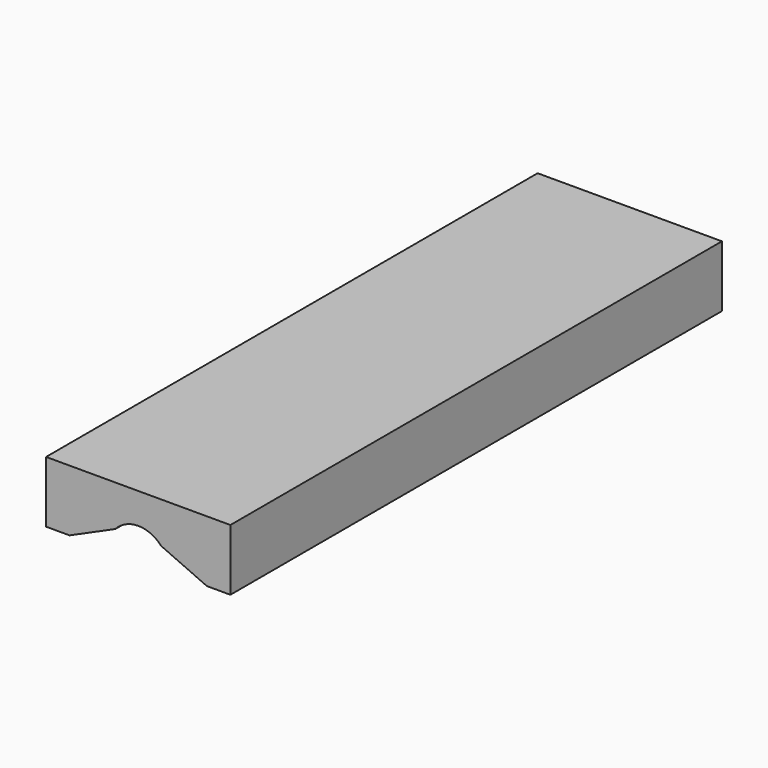
from build123d import *

# Parameters (mm, degrees)
F1_DEPTH    = 50
F2_T1_DEPTH = 66.3688124221


# Not quite as in the source:
# - a fillet or chamfer that OpenCascade refuses, or shapes differently, is made with other operations: its cross-section is extruded or revolved along the edge and cut away or added


with BuildPart() as f1:
    # F0 (on Front) → F1 (new body)
    with BuildSketch(Plane.XZ):
        with BuildLine():
            Line((7.5, 5), (0, 5))
            Line((0, 5), (-7.5, 5))
            Line((-7.5, 5), (-7.5, 0))
            Line((-7.5, 0), (-2.5, 0))
            ThreePointArc((-2.5, 0), (-1.767766953, 1.767766953), (0, 2.5))
            ThreePointArc((0, 2.5), (1.767766953, 1.767766953), (2.5, 0))
            Line((2.5, 0), (7.5, 0))
            Line((7.5, 0), (7.5, 5))
        make_face()
    extrude(amount=F1_DEPTH)

    # F2: chamfer of 5 on 2 edges, made by hand

    # F2_s2 → F2_t1 (cut)
    with BuildSketch(Plane.XZ.offset(-8.1844062111)):
        with BuildLine():
            Line((-5.5901699437, 0), (-1.8633899812, 1.6666666667))
            ThreePointArc((-1.8633899812, 1.6666666667), (-2.3064545677, 0.9645036688), (-2.5, 0))
            Line((-2.5, 0), (-5.5901699437, 0))
        make_face()
        with BuildLine():
            Line((5.5901699437, 0), (1.8633899812, 1.6666666667))
            ThreePointArc((1.8633899812, 1.6666666667), (2.3064545677, 0.9645036688), (2.5, 0))
            Line((2.5, 0), (5.5901699437, 0))
        make_face()
    extrude(amount=F2_T1_DEPTH, mode=Mode.SUBTRACT)


solid = f1.part
